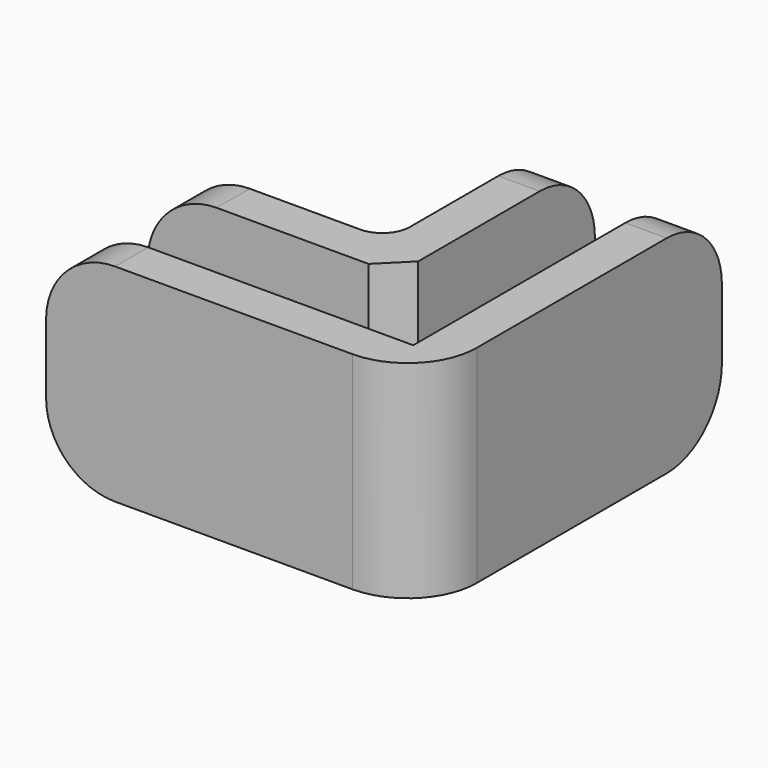
from build123d import *

# Parameters (mm, degrees)
F1_DEPTH     = 2
F2_DEPTH     = 15
F3_T1_DEPTH  = 28
F3_T3_DEPTH  = 28
F3_T5_DEPTH  = 28
F3_T7_DEPTH  = 28
F3_T9_DEPTH  = 37.2
F3_T11_DEPTH = 37.2
F3_T13_DEPTH = 40
F4_R         = 2
F5_SIZE      = 2


# Not quite as in the source:
# - a fillet or chamfer that OpenCascade refuses, or shapes differently, is made with other operations: its cross-section is extruded or revolved along the edge and cut away or added
# - a feature names something its author has since deleted; it is built from what else it names


with BuildPart() as f1:
    # F0 (on Top) → F1 (new body)
    with BuildSketch(Plane.XY):
        Polygon((0.9215265818, 0), (0.9215265818, 6.2), (0.9215265818, 24.2), (-5.2784734182, 24.2), (-5.2784734182, 6.2), (-23.2784734182, 6.2), (-23.2784734182, 0), (0, 0), align=None)
        Polygon((0.9215265818, 24.2), (0.9215265818, 6.2), (0.9215265818, 0), (0, 0), (-23.2784734182, 0), (-23.2784734182, -3), (0, -3), (3.9215265818, -3), (3.9215265818, 24.2), align=None)
        Polygon((-5.2784734182, 6.2), (-5.2784734182, 24.2), (-8.2784734182, 24.2), (-8.2784734182, 9.2), (-23.2784734182, 9.2), (-23.2784734182, 6.2), align=None)
    extrude(amount=F1_DEPTH)

    # F0 (on Top) → F2 (join)
    with BuildSketch(Plane.XY):
        Polygon((-5.2784734182, 6.2), (-5.2784734182, 24.2), (-8.2784734182, 24.2), (-8.2784734182, 9.2), (-23.2784734182, 9.2), (-23.2784734182, 6.2), align=None)
        Polygon((0.9215265818, 24.2), (0.9215265818, 6.2), (0.9215265818, 0), (0, 0), (-23.2784734182, 0), (-23.2784734182, -3), (0, -3), (3.9215265818, -3), (3.9215265818, 24.2), align=None)
    extrude(amount=F2_DEPTH)

    # F3: fillet of radius 5 on 7 edges, made by hand

    # F3_s2 → F3_t1 (cut)
    with BuildSketch(Plane.XZ.offset(-12.5)):
        with BuildLine():
            ThreePointArc((-18.2784734182, 15), (-21.8140073241, 13.5355339059), (-23.2784734182, 10))
            Line((-23.2784734182, 10), (-23.2784734182, 15))
            Line((-23.2784734182, 15), (-18.2784734182, 15))
        make_face()
    extrude(amount=F3_T1_DEPTH, mode=Mode.SUBTRACT)

    # F3_s4 → F3_t3 (cut)
    with BuildSketch(Plane.XZ.offset(-21.7)):
        with BuildLine():
            ThreePointArc((-18.2784734182, 15), (-21.8140073241, 13.5355339059), (-23.2784734182, 10))
            Line((-23.2784734182, 10), (-23.2784734182, 15))
            Line((-23.2784734182, 15), (-18.2784734182, 15))
        make_face()
    extrude(amount=F3_T3_DEPTH, mode=Mode.SUBTRACT)

    # F3_s6 → F3_t5 (cut)
    with BuildSketch(Plane.YZ.offset(-20.7784734182)):
        with BuildLine():
            ThreePointArc((19.2, 15), (22.7355339059, 13.5355339059), (24.2, 10))
            Line((24.2, 10), (24.2, 15))
            Line((24.2, 15), (19.2, 15))
        make_face()
    extrude(amount=F3_T5_DEPTH, mode=Mode.SUBTRACT)

    # F3_s8 → F3_t7 (cut)
    with BuildSketch(Plane.YZ.offset(-11.5784734182)):
        with BuildLine():
            ThreePointArc((24.2, 10), (22.7355339059, 13.5355339059), (19.2, 15))
            Line((19.2, 15), (24.2, 15))
            Line((24.2, 15), (24.2, 10))
        make_face()
    extrude(amount=F3_T7_DEPTH, mode=Mode.SUBTRACT)

    # F3_s10 → F3_t9 (cut)
    with BuildSketch(Plane.XZ.offset(-21.7)):
        with BuildLine():
            ThreePointArc((-18.2784734182, 0), (-21.8140073241, 1.4644660941), (-23.2784734182, 5))
            Line((-23.2784734182, 5), (-23.2784734182, 0))
            Line((-23.2784734182, 0), (-18.2784734182, 0))
        make_face()
    extrude(amount=F3_T9_DEPTH, mode=Mode.SUBTRACT)

    # F3_s12 → F3_t11 (cut)
    with BuildSketch(Plane.YZ.offset(-20.7784734182)):
        with BuildLine():
            ThreePointArc((19.2, 0), (22.7355339059, 1.4644660941), (24.2, 5))
            Line((24.2, 5), (24.2, 0))
            Line((24.2, 0), (19.2, 0))
        make_face()
    extrude(amount=F3_T11_DEPTH, mode=Mode.SUBTRACT)

    # F3_s14 → F3_t13 (cut)
    with BuildSketch(Plane.XY.offset(-12.5)):
        with BuildLine():
            ThreePointArc((-1.0784734182, -3), (2.4570604877, -1.5355339059), (3.9215265818, 2))
            Line((3.9215265818, 2), (3.9215265818, -3))
            Line((3.9215265818, -3), (-1.0784734182, -3))
        make_face()
    extrude(amount=F3_T13_DEPTH, mode=Mode.SUBTRACT)

    # F4
    f4_edges = [f1.edges().sort_by_distance(p)[0] for p in [
        (-8.278473, 9.2, 7.5),
    ]]
    fillet(f4_edges, radius=F4_R)

    # F5
    f5_edges = [f1.edges().sort_by_distance(p)[0] for p in [
        (-5.278473, 6.2, 8.5),
    ]]
    chamfer(f5_edges, length=F5_SIZE)


solid = f1.part
